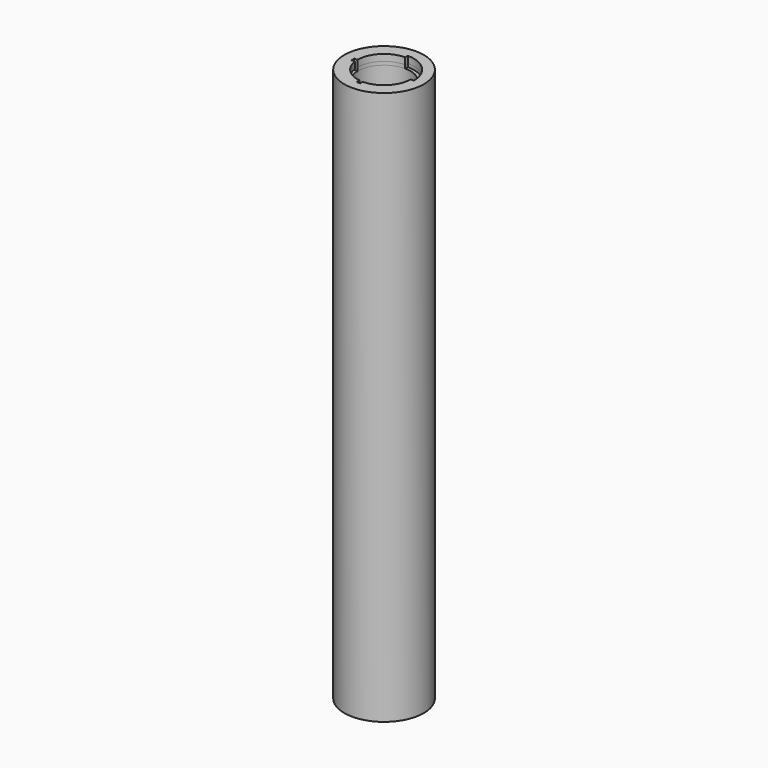
from build123d import *

# Parameters (mm, degrees)
F0_R     = 6
F1_DEPTH = 2.1
F2_R     = 6
F2_R_2   = 4
F3_DEPTH = 80
F4_R     = 6
F5_DEPTH = 0.5
F6_R     = 6
F7_DEPTH = 1


# Not quite as in the source:
# - after a boolean that leaves OpenCascade's solid faulty, fix() repairs it


with BuildPart() as f1:
    # F0 (on Top) → F1 (new body)
    with BuildSketch(Plane.XY):
        Circle(F0_R)
    extrude(amount=F1_DEPTH)

    # F2 (on face) → F3 (join)
    with BuildSketch(Plane.XY.offset(2.1)):
        Circle(F2_R)
        Circle(F2_R_2, mode=Mode.SUBTRACT)
    extrude(amount=F3_DEPTH)

    # F4 (on face) → F5 (join)
    with BuildSketch(Plane.XY.offset(82.1)):
        Circle(F4_R)
        with BuildLine():
            Line((0, 4), (0, 4.5))
            ThreePointArc((0, 4.5), (3.1819805153, 3.1819805153), (4.5, 0))
            Line((4.5, 0), (4, 0))
            ThreePointArc((4, 0), (2.8284271247, -2.8284271247), (0, -4))
            Line((0, -4), (0, -4.5))
            ThreePointArc((0, -4.5), (-3.1819805153, -3.1819805153), (-4.5, 0))
            Line((-4.5, 0), (-4, 0))
            ThreePointArc((-4, 0), (-2.8284271247, 2.8284271247), (0, 4))
        make_face(mode=Mode.SUBTRACT)
    extrude(amount=F5_DEPTH)

    add(f1.part.fix(), mode=Mode.REPLACE)

    # F6 (on face) → F7 (join)
    with BuildSketch(Plane.XY.offset(82.6)):
        Circle(F6_R)
        with BuildLine():
            ThreePointArc((-4, 0), (-2.8284271247, 2.8284271247), (0, 4))
            Line((0, 4), (0, 4.5))
            ThreePointArc((0, 4.5), (3.1819805153, 3.1819805153), (4.5, 0))
            Line((4.5, 0), (4, 0))
            ThreePointArc((4, 0), (2.8284271247, -2.8284271247), (0, -4))
            Line((0, -4), (0, -4.5))
            ThreePointArc((0, -4.5), (-0.2759966411, -4.4915282315), (-0.5509540913, -4.466144824))
            ThreePointArc((-0.5509540913, -4.466144824), (-3.1806256543, -3.1833347997), (-4.4656741218, -0.554756377))
            ThreePointArc((-4.4656741218, -0.554756377), (-4.4914103324, -0.2779086647), (-4.5, 0))
            Line((-4.5, 0), (-4, 0))
        make_face(mode=Mode.SUBTRACT)
        with BuildLine():
            ThreePointArc((-0.5509540913, -3.9618745045), (-2.8432495074, -2.813526655), (-3.9674454323, -0.5092904299))
            Line((-3.9674454323, -0.5092904299), (-4.4656741218, -0.554756377))
            ThreePointArc((-4.4656741218, -0.554756377), (-3.1806256543, -3.1833347997), (-0.5509540913, -4.466144824))
            Line((-0.5509540913, -4.466144824), (-0.5509540913, -3.9618745045))
        make_face()
    extrude(amount=F7_DEPTH)


solid = f1.part
